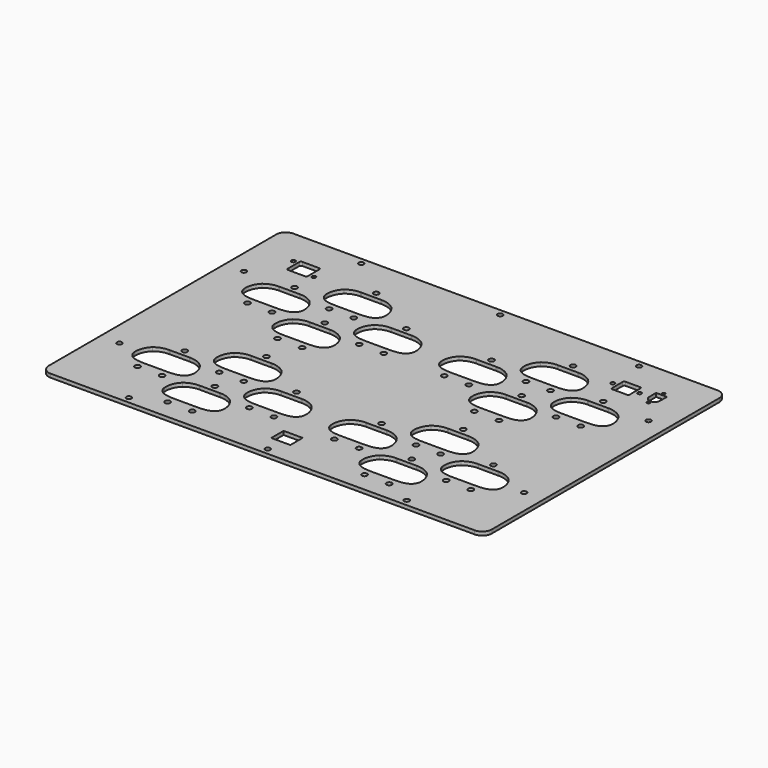
from build123d import *

# Parameters (mm, degrees)
F0_R     = 2.1
F0_R_2   = 2.2
F0_W     = 15.7
F0_H     = 12.7
F0_R_3   = 1.625
F0_R_4   = 1.6
F0_R_5   = 1.3
F1_DEPTH = 3


# Not quite as in the source:
# - the dataset's text gives a spline's control points without its knots; the knots are read off the source's solid


with BuildPart() as f1:
    # F0 (on Top) → F1 (new body)
    with BuildSketch(Plane.XY):
        with BuildLine():
            Line((174.5, 124.8), (-174.5, 124.8))
            ThreePointArc((-174.5, 124.8), (-180.0154328933, 122.5154328933), (-182.3, 117))
            Line((-182.3, 117), (-182.3, -117))
            ThreePointArc((-182.3, -117), (-180.0154328933, -122.5154328933), (-174.5, -124.8))
            Line((-174.5, -124.8), (174.5, -124.8))
            ThreePointArc((174.5, -124.8), (180.0154328933, -122.5154328933), (182.3, -117))
            Line((182.3, -117), (182.3, 117))
            ThreePointArc((182.3, 117), (180.0154328933, 122.5154328933), (174.5, 124.8))
        make_face()
        with Locations((-114.33, -119.5)):
            Circle(F0_R, mode=Mode.SUBTRACT)
        with Locations((-137.12, -82.102)):
            Circle(F0_R_2, mode=Mode.SUBTRACT)
        with Locations((-166.5, -64)):
            Circle(F0_R, mode=Mode.SUBTRACT)
        with Locations((-116.88, -82.102)):
            Circle(F0_R_2, mode=Mode.SUBTRACT)
        with BuildLine():
            Line((-135.6612948233, -51.451130735), (-135.115026498, -51.4620000001))
            Line((-135.115026498, -51.4620000001), (-118.8944121234, -51.4620000001))
            Line((-118.8944121234, -51.4620000001), (-118.3330315352, -51.4511211146))
            ThreePointArc((-118.3330315352, -51.4511211146), (-112.5954929046, -52.4136608229), (-107.487280821, -55.1979024679))
            ThreePointArc((-107.487280821, -55.1979024679), (-103.7289593809, -60.9649156398), (-102.7756384695, -67.7821438311))
            add(Edge.make_bspline(
                [(-102.7756384695, -67.7821438311), (-102.8317808557, -68.4791518436), (-103.1342622315, -69.8522558093), (-104.1227442667, -71.7376713061), (-105.3617732771, -73.0712234734), (-106.5853971676, -73.93803931), (-107.9464485907, -74.6539246569), (-109.8851336202, -75.2963766675), (-112.5588382079, -75.7473994177), (-115.5566427484, -75.9552688032), (-117.7556974045, -75.97825395), (-118.9009345935, -75.9720000001)],
                knots=[0, 0, 0, 0, 0.125, 0.25, 0.375, 0.4375, 0.5, 0.625, 0.75, 0.875, 0.9999501857, 0.9999501857, 0.9999501857, 0.9999501857], degree=3))
            Line((-118.9009345935, -75.9720000001), (-135.1072635354, -75.9720000001))
            Line((-135.1072635354, -75.9720000001), (-135.1086333173, -75.9720000001))
            add(Edge.make_bspline(
                [(-151.2339294072, -67.7821438309), (-151.177741554, -68.4797163167), (-150.8726831114, -69.8530561961), (-149.8774581613, -71.7367332364), (-148.6340002387, -73.0683891085), (-147.4094063644, -73.9344572306), (-146.0489657757, -74.6503376548), (-144.1131861346, -75.2935631846), (-141.4445788782, -75.7458922174), (-138.4515011772, -75.954911071), (-136.2539205452, -75.9782540848), (-135.1086333173, -75.9720000001)],
                knots=[0, 0, 0, 0, 0.125, 0.25, 0.375, 0.4375, 0.5, 0.625, 0.75, 0.875, 0.9999501867, 0.9999501867, 0.9999501867, 0.9999501867], degree=3))
            ThreePointArc((-151.2339294072, -67.7821438309), (-150.2806084958, -60.9649156397), (-146.5222870557, -55.1979024678))
            ThreePointArc((-146.5222870557, -55.1979024678), (-141.4068713777, -52.411174013), (-135.6612948233, -51.451130735))
        make_face(mode=Mode.SUBTRACT)
        with Locations((-91.12, -108.602)):
            Circle(F0_R_2, mode=Mode.SUBTRACT)
        with Locations((-70.88, -108.602)):
            Circle(F0_R_2, mode=Mode.SUBTRACT)
        with BuildLine():
            Line((-89.6612948233, -77.951130735), (-89.115026498, -77.9620000001))
            Line((-89.115026498, -77.9620000001), (-72.8944121234, -77.9620000001))
            Line((-72.8944121234, -77.9620000001), (-72.3330315352, -77.9511211146))
            ThreePointArc((-72.3330315352, -77.9511211146), (-66.5954929046, -78.9136608229), (-61.487280821, -81.6979024679))
            ThreePointArc((-61.487280821, -81.6979024679), (-57.7289593809, -87.4649156398), (-56.7756384695, -94.2821438311))
            add(Edge.make_bspline(
                [(-56.7756384695, -94.2821438311), (-56.8318288861, -94.9783630519), (-57.1341419789, -96.3506841544), (-58.1219861034, -98.2355446893), (-59.3608225377, -99.5692757568), (-60.5843212484, -100.4362682741), (-61.9452692843, -101.1523501476), (-63.8838615244, -101.7950820951), (-66.5575009571, -102.2464909201), (-69.5556737218, -102.4548208566), (-71.7552033004, -102.4781051534), (-72.9009345935, -102.4720000001)],
                knots=[0.0001387542, 0.0001387542, 0.0001387542, 0.0001387542, 0.125, 0.25, 0.375, 0.4375, 0.5, 0.625, 0.75, 0.875, 1, 1, 1, 1], degree=3))
            Line((-72.9009345935, -102.4720000001), (-89.1072635354, -102.4720000001))
            Line((-89.1072635354, -102.4720000001), (-89.1086333173, -102.4720000001))
            add(Edge.make_bspline(
                [(-105.2339294072, -94.2821438309), (-105.177741554, -94.9797163167), (-104.8726831114, -96.3530561961), (-103.8774581613, -98.2367332364), (-102.6340002387, -99.5683891085), (-101.4094063644, -100.4344572306), (-100.0489657757, -101.1503376548), (-98.1131861346, -101.7935631846), (-95.4445788782, -102.2458922174), (-92.4515011772, -102.454911071), (-90.2539205452, -102.4782540848), (-89.1086333173, -102.4720000001)],
                knots=[0, 0, 0, 0, 0.125, 0.25, 0.375, 0.4375, 0.5, 0.625, 0.75, 0.875, 0.9999501867, 0.9999501867, 0.9999501867, 0.9999501867], degree=3))
            ThreePointArc((-105.2339294072, -94.2821438309), (-104.2806084958, -87.4649156397), (-100.5222870557, -81.6979024678))
            ThreePointArc((-100.5222870557, -81.6979024678), (-95.4068713777, -78.911174013), (-89.6612948233, -77.951130735))
        make_face(mode=Mode.SUBTRACT)
        with Locations((-81, -72.692)):
            Circle(F0_R_2, mode=Mode.SUBTRACT)
        with Locations((-45.12, -82.102)):
            Circle(F0_R_2, mode=Mode.SUBTRACT)
        with Locations((-24.88, -82.102)):
            Circle(F0_R_2, mode=Mode.SUBTRACT)
        with BuildLine():
            Line((-43.6612948233, -51.451130735), (-43.115026498, -51.4620000001))
            Line((-43.115026498, -51.4620000001), (-26.8944121234, -51.4620000001))
            Line((-26.8944121234, -51.4620000001), (-26.3330315352, -51.4511211146))
            ThreePointArc((-26.3330315352, -51.4511211146), (-20.5954929046, -52.4136608229), (-15.487280821, -55.1979024679))
            ThreePointArc((-15.487280821, -55.1979024679), (-11.7289593809, -60.9649156398), (-10.7756384695, -67.7821438311))
            add(Edge.make_bspline(
                [(-10.7756384695, -67.7821438311), (-10.8317808557, -68.4791518436), (-11.1342622315, -69.8522558093), (-12.1227442667, -71.7376713061), (-13.3617732771, -73.0712234734), (-14.5853971676, -73.93803931), (-15.9464485907, -74.6539246569), (-17.8851336202, -75.2963766675), (-20.5588382079, -75.7473994177), (-23.5566427484, -75.9552688032), (-25.7556974045, -75.97825395), (-26.9009345935, -75.9720000001)],
                knots=[0, 0, 0, 0, 0.125, 0.25, 0.375, 0.4375, 0.5, 0.625, 0.75, 0.875, 0.9999501857, 0.9999501857, 0.9999501857, 0.9999501857], degree=3))
            Line((-26.9009345935, -75.9720000001), (-43.1072635354, -75.9720000001))
            Line((-43.1072635354, -75.9720000001), (-43.1086333173, -75.9720000001))
            add(Edge.make_bspline(
                [(-59.2339294072, -67.7821438309), (-59.177741554, -68.4797163167), (-58.8726831114, -69.8530561961), (-57.8774581613, -71.7367332364), (-56.6340002387, -73.0683891085), (-55.4094063644, -73.9344572306), (-54.0489657757, -74.6503376548), (-52.1131861346, -75.2935631846), (-49.4445788782, -75.7458922174), (-46.4515011772, -75.954911071), (-44.2539205452, -75.9782540848), (-43.1086333173, -75.9720000001)],
                knots=[0, 0, 0, 0, 0.125, 0.25, 0.375, 0.4375, 0.5, 0.625, 0.75, 0.875, 0.9999501867, 0.9999501867, 0.9999501867, 0.9999501867], degree=3))
            ThreePointArc((-59.2339294072, -67.7821438309), (-58.2806084958, -60.9649156397), (-54.5222870557, -55.1979024678))
            ThreePointArc((-54.5222870557, -55.1979024678), (-49.4068713777, -52.411174013), (-43.6612948233, -51.451130735))
        make_face(mode=Mode.SUBTRACT)
        with Locations((-127, -46.192)):
            Circle(F0_R_2, mode=Mode.SUBTRACT)
        with Locations((-91.12, -55.602)):
            Circle(F0_R_2, mode=Mode.SUBTRACT)
        with Locations((-70.88, -55.602)):
            Circle(F0_R_2, mode=Mode.SUBTRACT)
        with BuildLine():
            Line((-89.6612948233, -24.951130735), (-89.115026498, -24.9620000001))
            Line((-89.115026498, -24.9620000001), (-72.8944121234, -24.9620000001))
            Line((-72.8944121234, -24.9620000001), (-72.3330315352, -24.9511211146))
            ThreePointArc((-72.3330315352, -24.9511211146), (-66.5954929046, -25.9136608229), (-61.487280821, -28.6979024679))
            ThreePointArc((-61.487280821, -28.6979024679), (-57.7289593809, -34.4649156398), (-56.7756384695, -41.2821438311))
            add(Edge.make_bspline(
                [(-56.7756384695, -41.2821438311), (-56.8317808557, -41.9791518436), (-57.1342622315, -43.3522558093), (-58.1227442667, -45.2376713061), (-59.3617732771, -46.5712234734), (-60.5853971676, -47.43803931), (-61.9464485907, -48.1539246569), (-63.8851336202, -48.7963766675), (-66.5588382079, -49.2473994177), (-69.5566427484, -49.4552688032), (-71.7556974045, -49.47825395), (-72.9009345935, -49.4720000001)],
                knots=[0, 0, 0, 0, 0.125, 0.25, 0.375, 0.4375, 0.5, 0.625, 0.75, 0.875, 0.9999501857, 0.9999501857, 0.9999501857, 0.9999501857], degree=3))
            Line((-72.9009345935, -49.4720000001), (-89.1072635354, -49.4720000001))
            Line((-89.1072635354, -49.4720000001), (-89.1086333173, -49.4720000001))
            add(Edge.make_bspline(
                [(-105.2339294072, -41.2821438309), (-105.177741554, -41.9797163167), (-104.8726831114, -43.3530561961), (-103.8774581613, -45.2367332364), (-102.6340002387, -46.5683891085), (-101.4094063644, -47.4344572306), (-100.0489657757, -48.1503376548), (-98.1131861346, -48.7935631846), (-95.4445788782, -49.2458922174), (-92.4515011772, -49.454911071), (-90.2539205452, -49.4782540848), (-89.1086333173, -49.4720000001)],
                knots=[0, 0, 0, 0, 0.125, 0.25, 0.375, 0.4375, 0.5, 0.625, 0.75, 0.875, 0.9999501867, 0.9999501867, 0.9999501867, 0.9999501867], degree=3))
            ThreePointArc((-105.2339294072, -41.2821438309), (-104.2806084958, -34.4649156397), (-100.5222870557, -28.6979024678))
            ThreePointArc((-100.5222870557, -28.6979024678), (-95.4068713777, -25.911174013), (-89.6612948233, -24.951130735))
        make_face(mode=Mode.SUBTRACT)
        with Locations((-35, -46.192)):
            Circle(F0_R_2, mode=Mode.SUBTRACT)
        with Locations((-81, -19.692)):
            Circle(F0_R_2, mode=Mode.SUBTRACT)
        with Locations((0, -119.5)):
            Circle(F0_R, mode=Mode.SUBTRACT)
        with Locations((0, -99.8)):
            Rectangle(F0_W, F0_H, mode=Mode.SUBTRACT)
        with Locations((70.88, -108.602)):
            Circle(F0_R_2, mode=Mode.SUBTRACT)
        with Locations((91.12, -108.602)):
            Circle(F0_R_2, mode=Mode.SUBTRACT)
        with Locations((24.88, -82.102)):
            Circle(F0_R_2, mode=Mode.SUBTRACT)
        with Locations((45.12, -82.102)):
            Circle(F0_R_2, mode=Mode.SUBTRACT)
        with BuildLine():
            Line((26.3387051767, -51.451130735), (26.884973502, -51.4620000001))
            Line((26.884973502, -51.4620000001), (43.1055878766, -51.4620000001))
            Line((43.1055878766, -51.4620000001), (43.6669684648, -51.4511211146))
            ThreePointArc((43.6669684648, -51.4511211146), (49.4045070954, -52.4136608229), (54.512719179, -55.1979024679))
            ThreePointArc((54.512719179, -55.1979024679), (58.2710406191, -60.9649156398), (59.2243615305, -67.7821438311))
            add(Edge.make_bspline(
                [(59.2243615305, -67.7821438311), (59.1682191443, -68.4791518436), (58.8657377685, -69.8522558093), (57.8772557333, -71.7376713061), (56.6382267229, -73.0712234734), (55.4146028324, -73.93803931), (54.0535514093, -74.6539246569), (52.1148663798, -75.2963766675), (49.4411617921, -75.7473994177), (46.4433572516, -75.9552688032), (44.2443025955, -75.97825395), (43.0990654065, -75.9720000001)],
                knots=[0, 0, 0, 0, 0.125, 0.25, 0.375, 0.4375, 0.5, 0.625, 0.75, 0.875, 0.9999501857, 0.9999501857, 0.9999501857, 0.9999501857], degree=3))
            Line((43.0990654065, -75.9720000001), (26.8927364646, -75.9720000001))
            Line((26.8927364646, -75.9720000001), (26.8913666827, -75.9720000001))
            add(Edge.make_bspline(
                [(10.7660705928, -67.7821438309), (10.822258446, -68.4797163167), (11.1273168886, -69.8530561961), (12.1225418387, -71.7367332364), (13.3659997613, -73.0683891085), (14.5905936356, -73.9344572306), (15.9510342243, -74.6503376548), (17.8868138654, -75.2935631846), (20.5554211218, -75.7458922174), (23.5484988228, -75.954911071), (25.7460794548, -75.9782540848), (26.8913666827, -75.9720000001)],
                knots=[0, 0, 0, 0, 0.125, 0.25, 0.375, 0.4375, 0.5, 0.625, 0.75, 0.875, 0.9999501867, 0.9999501867, 0.9999501867, 0.9999501867], degree=3))
            ThreePointArc((10.7660705928, -67.7821438309), (11.7193915042, -60.9649156397), (15.4777129443, -55.1979024678))
            ThreePointArc((15.4777129443, -55.1979024678), (20.5931286223, -52.411174013), (26.3387051767, -51.451130735))
        make_face(mode=Mode.SUBTRACT)
        with BuildLine():
            Line((72.3387051767, -77.951130735), (72.884973502, -77.9620000001))
            Line((72.884973502, -77.9620000001), (89.1055878766, -77.9620000001))
            Line((89.1055878766, -77.9620000001), (89.6669684648, -77.9511211146))
            ThreePointArc((89.6669684648, -77.9511211146), (95.4045070954, -78.9136608229), (100.512719179, -81.6979024679))
            ThreePointArc((100.512719179, -81.6979024679), (104.2710406191, -87.4649156398), (105.2243615305, -94.2821438311))
            add(Edge.make_bspline(
                [(105.2243615305, -94.2821438311), (105.1682191443, -94.9791518436), (104.8657377685, -96.3522558093), (103.8772557333, -98.2376713061), (102.6382267229, -99.5712234734), (101.4146028324, -100.43803931), (100.0535514093, -101.1539246569), (98.1148663798, -101.7963766675), (95.4411617921, -102.2473994177), (92.4433572516, -102.4552688032), (90.2443025955, -102.47825395), (89.0990654065, -102.4720000001)],
                knots=[0, 0, 0, 0, 0.125, 0.25, 0.375, 0.4375, 0.5, 0.625, 0.75, 0.875, 0.9999501857, 0.9999501857, 0.9999501857, 0.9999501857], degree=3))
            Line((89.0990654065, -102.4720000001), (72.8927364646, -102.4720000001))
            Line((72.8927364646, -102.4720000001), (72.8913666827, -102.4720000001))
            add(Edge.make_bspline(
                [(56.7660705928, -94.2821438309), (56.822258446, -94.9797163167), (57.1273168886, -96.3530561961), (58.1225418387, -98.2367332364), (59.3659997613, -99.5683891085), (60.5905936356, -100.4344572306), (61.9510342243, -101.1503376548), (63.8868138654, -101.7935631846), (66.5554211218, -102.2458922174), (69.5484988228, -102.454911071), (71.7460794548, -102.4782540848), (72.8913666827, -102.4720000001)],
                knots=[0, 0, 0, 0, 0.125, 0.25, 0.375, 0.4375, 0.5, 0.625, 0.75, 0.875, 0.9999501867, 0.9999501867, 0.9999501867, 0.9999501867], degree=3))
            ThreePointArc((56.7660705928, -94.2821438309), (57.7193915042, -87.4649156397), (61.4777129443, -81.6979024678))
            ThreePointArc((61.4777129443, -81.6979024678), (66.5931286223, -78.911174013), (72.3387051767, -77.951130735))
        make_face(mode=Mode.SUBTRACT)
        with Locations((81, -72.692)):
            Circle(F0_R_2, mode=Mode.SUBTRACT)
        with Locations((114.33, -119.5)):
            Circle(F0_R, mode=Mode.SUBTRACT)
        with Locations((116.88, -82.102)):
            Circle(F0_R_2, mode=Mode.SUBTRACT)
        with BuildLine():
            Line((118.3387051767, -51.451130735), (118.884973502, -51.4620000001))
            Line((118.884973502, -51.4620000001), (135.1055878766, -51.4620000001))
            Line((135.1055878766, -51.4620000001), (135.6669684648, -51.4511211146))
            ThreePointArc((135.6669684648, -51.4511211146), (141.4045070954, -52.4136608229), (146.512719179, -55.1979024679))
            ThreePointArc((146.512719179, -55.1979024679), (150.2710406191, -60.9649156398), (151.2243615305, -67.7821438311))
            add(Edge.make_bspline(
                [(151.2243615305, -67.7821438311), (151.1682191443, -68.4791518436), (150.8657377685, -69.8522558093), (149.8772557333, -71.7376713061), (148.6382267229, -73.0712234734), (147.4146028324, -73.93803931), (146.0535514093, -74.6539246569), (144.1148663798, -75.2963766675), (141.4411617921, -75.7473994177), (138.4433572516, -75.9552688032), (136.2443025955, -75.97825395), (135.0990654065, -75.9720000001)],
                knots=[0, 0, 0, 0, 0.125, 0.25, 0.375, 0.4375, 0.5, 0.625, 0.75, 0.875, 0.9999501857, 0.9999501857, 0.9999501857, 0.9999501857], degree=3))
            Line((135.0990654065, -75.9720000001), (118.8927364646, -75.9720000001))
            Line((118.8927364646, -75.9720000001), (118.8913666827, -75.9720000001))
            add(Edge.make_bspline(
                [(102.7660705928, -67.7821438309), (102.822258446, -68.4797163167), (103.1273168886, -69.8530561961), (104.1225418387, -71.7367332364), (105.3659997613, -73.0683891085), (106.5905936356, -73.9344572306), (107.9510342243, -74.6503376548), (109.8868138654, -75.2935631846), (112.5554211218, -75.7458922174), (115.5484988228, -75.954911071), (117.7460794548, -75.9782540848), (118.8913666827, -75.9720000001)],
                knots=[0, 0, 0, 0, 0.125, 0.25, 0.375, 0.4375, 0.5, 0.625, 0.75, 0.875, 0.9999501867, 0.9999501867, 0.9999501867, 0.9999501867], degree=3))
            ThreePointArc((102.7660705928, -67.7821438309), (103.7193915042, -60.9649156397), (107.4777129443, -55.1979024678))
            ThreePointArc((107.4777129443, -55.1979024678), (112.5931286223, -52.411174013), (118.3387051767, -51.451130735))
        make_face(mode=Mode.SUBTRACT)
        with Locations((137.12, -82.102)):
            Circle(F0_R_2, mode=Mode.SUBTRACT)
        with Locations((166.5, -64)):
            Circle(F0_R, mode=Mode.SUBTRACT)
        with Locations((35, -46.192)):
            Circle(F0_R_2, mode=Mode.SUBTRACT)
        with Locations((70.88, -55.602)):
            Circle(F0_R_2, mode=Mode.SUBTRACT)
        with Locations((91.12, -55.602)):
            Circle(F0_R_2, mode=Mode.SUBTRACT)
        with BuildLine():
            Line((72.3387051767, -24.951130735), (72.884973502, -24.9620000001))
            Line((72.884973502, -24.9620000001), (89.1055878766, -24.9620000001))
            Line((89.1055878766, -24.9620000001), (89.6669684648, -24.9511211146))
            ThreePointArc((89.6669684648, -24.9511211146), (95.4045070954, -25.9136608229), (100.512719179, -28.6979024679))
            ThreePointArc((100.512719179, -28.6979024679), (104.2710406191, -34.4649156398), (105.2243615305, -41.2821438311))
            add(Edge.make_bspline(
                [(105.2243615305, -41.2821438311), (105.1682191443, -41.9791518436), (104.8657377685, -43.3522558093), (103.8772557333, -45.2376713061), (102.6382267229, -46.5712234734), (101.4146028324, -47.43803931), (100.0535514093, -48.1539246569), (98.1148663798, -48.7963766675), (95.4411617921, -49.2473994177), (92.4433572516, -49.4552688032), (90.2443025955, -49.47825395), (89.0990654065, -49.4720000001)],
                knots=[0, 0, 0, 0, 0.125, 0.25, 0.375, 0.4375, 0.5, 0.625, 0.75, 0.875, 0.9999501857, 0.9999501857, 0.9999501857, 0.9999501857], degree=3))
            Line((89.0990654065, -49.4720000001), (72.8927364646, -49.4720000001))
            Line((72.8927364646, -49.4720000001), (72.8913666827, -49.4720000001))
            add(Edge.make_bspline(
                [(56.7660705928, -41.2821438309), (56.822258446, -41.9797163167), (57.1273168886, -43.3530561961), (58.1225418387, -45.2367332364), (59.3659997613, -46.5683891085), (60.5905936356, -47.4344572306), (61.9510342243, -48.1503376548), (63.8868138654, -48.7935631846), (66.5554211218, -49.2458922174), (69.5484988228, -49.454911071), (71.7460794548, -49.4782540848), (72.8913666827, -49.4720000001)],
                knots=[0, 0, 0, 0, 0.125, 0.25, 0.375, 0.4375, 0.5, 0.625, 0.75, 0.875, 0.9999501867, 0.9999501867, 0.9999501867, 0.9999501867], degree=3))
            ThreePointArc((56.7660705928, -41.2821438309), (57.7193915042, -34.4649156397), (61.4777129443, -28.6979024678))
            ThreePointArc((61.4777129443, -28.6979024678), (66.5931286223, -25.911174013), (72.3387051767, -24.951130735))
        make_face(mode=Mode.SUBTRACT)
        with Locations((81, -19.692)):
            Circle(F0_R_2, mode=Mode.SUBTRACT)
        with Locations((127, -46.192)):
            Circle(F0_R_2, mode=Mode.SUBTRACT)
        with Locations((-137.12, 30.898)):
            Circle(F0_R_2, mode=Mode.SUBTRACT)
        with Locations((-116.88, 30.898)):
            Circle(F0_R_2, mode=Mode.SUBTRACT)
        with BuildLine():
            Line((-135.6612948233, 61.548869265), (-135.115026498, 61.5379999999))
            Line((-135.115026498, 61.5379999999), (-118.8944121234, 61.5379999999))
            Line((-118.8944121234, 61.5379999999), (-118.3330315352, 61.5488788854))
            ThreePointArc((-118.3330315352, 61.5488788854), (-112.5954929046, 60.5863391771), (-107.487280821, 57.8020975321))
            ThreePointArc((-107.487280821, 57.8020975321), (-103.7289593809, 52.0350843602), (-102.7756384695, 45.2178561689))
            add(Edge.make_bspline(
                [(-102.7756384695, 45.2178561689), (-102.8317808557, 44.5208481564), (-103.1342622315, 43.1477441907), (-104.1227442667, 41.2623286939), (-105.3617732771, 39.9287765266), (-106.5853971676, 39.06196069), (-107.9464485907, 38.3460753431), (-109.8851336202, 37.7036233325), (-112.5588382079, 37.2526005823), (-115.5566427484, 37.0447311968), (-117.7556974045, 37.02174605), (-118.9009345935, 37.0279999999)],
                knots=[0, 0, 0, 0, 0.125, 0.25, 0.375, 0.4375, 0.5, 0.625, 0.75, 0.875, 0.9999501857, 0.9999501857, 0.9999501857, 0.9999501857], degree=3))
            Line((-118.9009345935, 37.0279999999), (-135.1072635354, 37.0279999999))
            Line((-135.1072635354, 37.0279999999), (-135.1086333173, 37.0279999999))
            add(Edge.make_bspline(
                [(-151.2339294072, 45.2178561691), (-151.177741554, 44.5202836833), (-150.8726831114, 43.1469438039), (-149.8774581613, 41.2632667636), (-148.6340002387, 39.9316108915), (-147.4094063644, 39.0655427694), (-146.0489657757, 38.3496623452), (-144.1131861346, 37.7064368154), (-141.4445788782, 37.2541077826), (-138.4515011772, 37.045088929), (-136.2539205452, 37.0217459152), (-135.1086333173, 37.0279999999)],
                knots=[0, 0, 0, 0, 0.125, 0.25, 0.375, 0.4375, 0.5, 0.625, 0.75, 0.875, 0.9999501867, 0.9999501867, 0.9999501867, 0.9999501867], degree=3))
            ThreePointArc((-151.2339294072, 45.2178561691), (-150.2806084958, 52.0350843603), (-146.5222870557, 57.8020975322))
            ThreePointArc((-146.5222870557, 57.8020975322), (-141.4068713777, 60.588825987), (-135.6612948233, 61.548869265))
        make_face(mode=Mode.SUBTRACT)
        with Locations((-91.12, 4.398)):
            Circle(F0_R_2, mode=Mode.SUBTRACT)
        with Locations((-70.88, 4.398)):
            Circle(F0_R_2, mode=Mode.SUBTRACT)
        with BuildLine():
            Line((-89.6612948233, 35.048869265), (-89.115026498, 35.0379999999))
            Line((-89.115026498, 35.0379999999), (-72.8944121234, 35.0379999999))
            Line((-72.8944121234, 35.0379999999), (-72.3330315352, 35.0488788854))
            ThreePointArc((-72.3330315352, 35.0488788854), (-66.5954929046, 34.0863391771), (-61.487280821, 31.3020975321))
            ThreePointArc((-61.487280821, 31.3020975321), (-57.7289593809, 25.5350843602), (-56.7756384695, 18.7178561689))
            add(Edge.make_bspline(
                [(-56.7756384695, 18.7178561689), (-56.8317808557, 18.0208481564), (-57.1342622315, 16.6477441907), (-58.1227442667, 14.7623286939), (-59.3617732771, 13.4287765266), (-60.5853971676, 12.56196069), (-61.9464485907, 11.8460753431), (-63.8851336202, 11.2036233325), (-66.5588382079, 10.7526005823), (-69.5566427484, 10.5447311968), (-71.7556974045, 10.52174605), (-72.9009345935, 10.5279999999)],
                knots=[0, 0, 0, 0, 0.125, 0.25, 0.375, 0.4375, 0.5, 0.625, 0.75, 0.875, 0.9999501857, 0.9999501857, 0.9999501857, 0.9999501857], degree=3))
            Line((-72.9009345935, 10.5279999999), (-89.1072635354, 10.5279999999))
            Line((-89.1072635354, 10.5279999999), (-89.1086333173, 10.5279999999))
            add(Edge.make_bspline(
                [(-105.2339294072, 18.7178561691), (-105.177741554, 18.0202836833), (-104.8726831114, 16.6469438039), (-103.8774581613, 14.7632667636), (-102.6340002387, 13.4316108915), (-101.4094063644, 12.5655427694), (-100.0489657757, 11.8496623452), (-98.1131861346, 11.2064368154), (-95.4445788782, 10.7541077826), (-92.4515011772, 10.545088929), (-90.2539205452, 10.5217459152), (-89.1086333173, 10.5279999999)],
                knots=[0, 0, 0, 0, 0.125, 0.25, 0.375, 0.4375, 0.5, 0.625, 0.75, 0.875, 0.9999501867, 0.9999501867, 0.9999501867, 0.9999501867], degree=3))
            ThreePointArc((-105.2339294072, 18.7178561691), (-104.2806084958, 25.5350843603), (-100.5222870557, 31.3020975322))
            ThreePointArc((-100.5222870557, 31.3020975322), (-95.4068713777, 34.088825987), (-89.6612948233, 35.048869265))
        make_face(mode=Mode.SUBTRACT)
        with Locations((-45.12, 30.898)):
            Circle(F0_R_2, mode=Mode.SUBTRACT)
        with Locations((-24.88, 30.898)):
            Circle(F0_R_2, mode=Mode.SUBTRACT)
        with Locations((-81, 40.308)):
            Circle(F0_R_2, mode=Mode.SUBTRACT)
        with Locations((-91.12, 57.398)):
            Circle(F0_R_2, mode=Mode.SUBTRACT)
        with Locations((-70.88, 57.398)):
            Circle(F0_R_2, mode=Mode.SUBTRACT)
        with BuildLine():
            Line((-43.6612948233, 61.548869265), (-43.115026498, 61.5379999999))
            Line((-43.115026498, 61.5379999999), (-26.8944121234, 61.5379999999))
            Line((-26.8944121234, 61.5379999999), (-26.3330315352, 61.5488788854))
            ThreePointArc((-26.3330315352, 61.5488788854), (-20.5954929046, 60.5863391771), (-15.487280821, 57.8020975321))
            ThreePointArc((-15.487280821, 57.8020975321), (-11.7282191214, 52.0352577574), (-10.7742686876, 45.2178561689))
            add(Edge.make_bspline(
                [(-10.7742686876, 45.2178561689), (-10.8304110738, 44.5208481564), (-11.1328924496, 43.1477441907), (-12.1213744847, 41.2623286939), (-13.3604034952, 39.9287765266), (-14.5840273857, 39.06196069), (-15.9450788087, 38.3460753431), (-17.8837638383, 37.7036233325), (-20.557468426, 37.2526005823), (-23.5552729664, 37.0447311968), (-25.7543276226, 37.02174605), (-26.8995648116, 37.0279999999)],
                knots=[0, 0, 0, 0, 0.125, 0.25, 0.375, 0.4375, 0.5, 0.625, 0.75, 0.875, 0.9999501857, 0.9999501857, 0.9999501857, 0.9999501857], degree=3))
            Line((-26.8995648116, 37.0279999999), (-43.1072635354, 37.0279999999))
            add(Edge.make_bspline(
                [(-59.2325596253, 45.2178561691), (-59.1763212388, 44.5210734563), (-58.8714315071, 43.1485163208), (-57.876846428, 41.2653920745), (-56.633580812, 39.9335566586), (-55.4091120122, 39.0673117119), (-54.0487748122, 38.3512348451), (-52.1130880742, 37.7077297918), (-49.4445461628, 37.255015412), (-46.4511010398, 37.0455365283), (-44.2530455057, 37.0218945801), (-43.1072635354, 37.0279999999)],
                knots=[0.0001386451, 0.0001386451, 0.0001386451, 0.0001386451, 0.125, 0.25, 0.375, 0.4375, 0.5, 0.625, 0.75, 0.875, 1, 1, 1, 1], degree=3))
            ThreePointArc((-59.2325596253, 45.2178561691), (-58.2798682404, 52.0349109767), (-54.5222870557, 57.8020975322))
            ThreePointArc((-54.5222870557, 57.8020975322), (-49.4068713777, 60.588825987), (-43.6612948233, 61.548869265))
        make_face(mode=Mode.SUBTRACT)
        with Locations((-166.5, 64)):
            Circle(F0_R, mode=Mode.SUBTRACT)
        with BuildLine():
            ThreePointArc((-146.775, 96.295), (-146.370807358, 97.270807358), (-145.395, 97.675))
            Line((-145.395, 97.675), (-131.605, 97.675))
            ThreePointArc((-131.605, 97.675), (-130.629192642, 97.270807358), (-130.225, 96.295))
            Line((-130.225, 96.295), (-130.225, 84.505))
            ThreePointArc((-130.225, 84.505), (-130.629192642, 83.529192642), (-131.605, 83.125))
            Line((-131.605, 83.125), (-145.395, 83.125))
            ThreePointArc((-145.395, 83.125), (-146.370807358, 83.529192642), (-146.775, 84.505))
            Line((-146.775, 84.505), (-146.775, 96.295))
        make_face(mode=Mode.SUBTRACT)
        with Locations((-127, 66.808)):
            Circle(F0_R_2, mode=Mode.SUBTRACT)
        with Locations((-126.5, 85.9)):
            Circle(F0_R_3, mode=Mode.SUBTRACT)
        with Locations((-150.5, 94.9)):
            Circle(F0_R_3, mode=Mode.SUBTRACT)
        with Locations((-114.33, 119.5)):
            Circle(F0_R, mode=Mode.SUBTRACT)
        with BuildLine():
            Line((-89.6612948233, 88.048869265), (-89.115026498, 88.0379999999))
            Line((-89.115026498, 88.0379999999), (-72.8944121234, 88.0379999999))
            Line((-72.8944121234, 88.0379999999), (-72.3330315352, 88.0488788854))
            ThreePointArc((-72.3330315352, 88.0488788854), (-66.5954929046, 87.0863391771), (-61.487280821, 84.3020975321))
            ThreePointArc((-61.487280821, 84.3020975321), (-57.7289593809, 78.5350843602), (-56.7756384695, 71.7178561689))
            add(Edge.make_bspline(
                [(-56.7756384695, 71.7178561689), (-56.8317808557, 71.0208481564), (-57.1342622315, 69.6477441907), (-58.1227442667, 67.7623286939), (-59.3617732771, 66.4287765266), (-60.5853971676, 65.56196069), (-61.9464485907, 64.8460753431), (-63.8851336202, 64.2036233325), (-66.5588382079, 63.7526005823), (-69.5566427484, 63.5447311968), (-71.7556974045, 63.52174605), (-72.9009345935, 63.5279999999)],
                knots=[0, 0, 0, 0, 0.125, 0.25, 0.375, 0.4375, 0.5, 0.625, 0.75, 0.875, 0.9999501857, 0.9999501857, 0.9999501857, 0.9999501857], degree=3))
            Line((-72.9009345935, 63.5279999999), (-89.1072635354, 63.5279999999))
            Line((-89.1072635354, 63.5279999999), (-89.1086333173, 63.5279999999))
            add(Edge.make_bspline(
                [(-105.2339294072, 71.7178561691), (-105.177741554, 71.0202836833), (-104.8726831114, 69.6469438039), (-103.8774581613, 67.7632667636), (-102.6340002387, 66.4316108915), (-101.4094063644, 65.5655427694), (-100.0489657757, 64.8496623452), (-98.1131861346, 64.2064368154), (-95.4445788782, 63.7541077826), (-92.4515011772, 63.545088929), (-90.2539205452, 63.5217459152), (-89.1086333173, 63.5279999999)],
                knots=[0, 0, 0, 0, 0.125, 0.25, 0.375, 0.4375, 0.5, 0.625, 0.75, 0.875, 0.9999501867, 0.9999501867, 0.9999501867, 0.9999501867], degree=3))
            ThreePointArc((-105.2339294072, 71.7178561691), (-104.2806084958, 78.5350843603), (-100.5222870557, 84.3020975322))
            ThreePointArc((-100.5222870557, 84.3020975322), (-95.4068713777, 87.088825987), (-89.6612948233, 88.048869265))
        make_face(mode=Mode.SUBTRACT)
        with Locations((-81, 93.308)):
            Circle(F0_R_2, mode=Mode.SUBTRACT)
        with Locations((-35, 66.808)):
            Circle(F0_R_2, mode=Mode.SUBTRACT)
        with Locations((24.88, 30.898)):
            Circle(F0_R_2, mode=Mode.SUBTRACT)
        with Locations((45.12, 30.898)):
            Circle(F0_R_2, mode=Mode.SUBTRACT)
        with Locations((70.88, 4.398)):
            Circle(F0_R_2, mode=Mode.SUBTRACT)
        with Locations((91.12, 4.398)):
            Circle(F0_R_2, mode=Mode.SUBTRACT)
        with BuildLine():
            Line((72.3387051767, 35.048869265), (72.884973502, 35.0379999999))
            Line((72.884973502, 35.0379999999), (89.1055878766, 35.0379999999))
            Line((89.1055878766, 35.0379999999), (89.6669684648, 35.0488788854))
            ThreePointArc((89.6669684648, 35.0488788854), (95.4045070954, 34.0863391771), (100.512719179, 31.3020975321))
            ThreePointArc((100.512719179, 31.3020975321), (104.2710406191, 25.5350843602), (105.2243615305, 18.7178561689))
            add(Edge.make_bspline(
                [(105.2243615305, 18.7178561689), (105.1681711139, 18.0216369481), (104.8658580211, 16.6493158456), (103.8780138966, 14.7644553107), (102.6391774623, 13.4307242432), (101.4156787516, 12.5637317259), (100.0547307157, 11.8476498524), (98.1161384756, 11.2049179049), (95.4424990429, 10.7535090799), (92.4443262782, 10.5451791434), (90.2447966996, 10.5218948466), (89.0990654065, 10.5279999999)],
                knots=[0.0001387542, 0.0001387542, 0.0001387542, 0.0001387542, 0.125, 0.25, 0.375, 0.4375, 0.5, 0.625, 0.75, 0.875, 1, 1, 1, 1], degree=3))
            Line((89.0990654065, 10.5279999999), (72.8927364646, 10.5279999999))
            Line((72.8927364646, 10.5279999999), (72.8913666827, 10.5279999999))
            add(Edge.make_bspline(
                [(56.7660705928, 18.7178561691), (56.822258446, 18.0202836833), (57.1273168886, 16.6469438039), (58.1225418387, 14.7632667636), (59.3659997613, 13.4316108915), (60.5905936356, 12.5655427694), (61.9510342243, 11.8496623452), (63.8868138654, 11.2064368154), (66.5554211218, 10.7541077826), (69.5484988228, 10.545088929), (71.7460794548, 10.5217459152), (72.8913666827, 10.5279999999)],
                knots=[0, 0, 0, 0, 0.125, 0.25, 0.375, 0.4375, 0.5, 0.625, 0.75, 0.875, 0.9999501867, 0.9999501867, 0.9999501867, 0.9999501867], degree=3))
            ThreePointArc((56.7660705928, 18.7178561691), (57.7193915042, 25.5350843603), (61.4777129443, 31.3020975322))
            ThreePointArc((61.4777129443, 31.3020975322), (66.5931286223, 34.088825987), (72.3387051767, 35.048869265))
        make_face(mode=Mode.SUBTRACT)
        with BuildLine():
            Line((26.3387051767, 61.548869265), (26.884973502, 61.5379999999))
            Line((26.884973502, 61.5379999999), (43.1055878766, 61.5379999999))
            Line((43.1055878766, 61.5379999999), (43.6669684648, 61.5488788854))
            ThreePointArc((43.6669684648, 61.5488788854), (49.4045070954, 60.5863391771), (54.512719179, 57.8020975321))
            ThreePointArc((54.512719179, 57.8020975321), (58.2710406191, 52.0350843602), (59.2243615305, 45.2178561689))
            add(Edge.make_bspline(
                [(59.2243615305, 45.2178561689), (59.1681711139, 44.5216369481), (58.8658580211, 43.1493158456), (57.8780138966, 41.2644553107), (56.6391774623, 39.9307242432), (55.4156787516, 39.0637317259), (54.0547307157, 38.3476498524), (52.1161384756, 37.7049179049), (49.4424990429, 37.2535090799), (46.4443262782, 37.0451791434), (44.2447966996, 37.0218948466), (43.0990654065, 37.0279999999)],
                knots=[0.0001387542, 0.0001387542, 0.0001387542, 0.0001387542, 0.125, 0.25, 0.375, 0.4375, 0.5, 0.625, 0.75, 0.875, 1, 1, 1, 1], degree=3))
            Line((43.0990654065, 37.0279999999), (26.8927364646, 37.0279999999))
            Line((26.8927364646, 37.0279999999), (26.8913666827, 37.0279999999))
            add(Edge.make_bspline(
                [(10.7660705928, 45.2178561691), (10.822258446, 44.5202836833), (11.1273168886, 43.1469438039), (12.1225418387, 41.2632667636), (13.3659997613, 39.9316108915), (14.5905936356, 39.0655427694), (15.9510342243, 38.3496623452), (17.8868138654, 37.7064368154), (20.5554211218, 37.2541077826), (23.5484988228, 37.045088929), (25.7460794548, 37.0217459152), (26.8913666827, 37.0279999999)],
                knots=[0, 0, 0, 0, 0.125, 0.25, 0.375, 0.4375, 0.5, 0.625, 0.75, 0.875, 0.9999501867, 0.9999501867, 0.9999501867, 0.9999501867], degree=3))
            ThreePointArc((10.7660705928, 45.2178561691), (11.7193915042, 52.0350843603), (15.4777129443, 57.8020975322))
            ThreePointArc((15.4777129443, 57.8020975322), (20.5931286223, 60.588825987), (26.3387051767, 61.548869265))
        make_face(mode=Mode.SUBTRACT)
        with Locations((81, 40.308)):
            Circle(F0_R_2, mode=Mode.SUBTRACT)
        with Locations((70.88, 57.398)):
            Circle(F0_R_2, mode=Mode.SUBTRACT)
        with Locations((91.12, 57.398)):
            Circle(F0_R_2, mode=Mode.SUBTRACT)
        with Locations((116.88, 30.898)):
            Circle(F0_R_2, mode=Mode.SUBTRACT)
        with Locations((137.12, 30.898)):
            Circle(F0_R_2, mode=Mode.SUBTRACT)
        with BuildLine():
            Line((118.3387051767, 61.548869265), (118.884973502, 61.5379999999))
            Line((118.884973502, 61.5379999999), (135.1055878766, 61.5379999999))
            Line((135.1055878766, 61.5379999999), (135.6669684648, 61.5488788854))
            ThreePointArc((135.6669684648, 61.5488788854), (141.4045070954, 60.5863391771), (146.512719179, 57.8020975321))
            ThreePointArc((146.512719179, 57.8020975321), (150.2710406191, 52.0350843602), (151.2243615305, 45.2178561689))
            add(Edge.make_bspline(
                [(151.2243615305, 45.2178561689), (151.1681711139, 44.5216369481), (150.8658580211, 43.1493158456), (149.8780138966, 41.2644553107), (148.6391774623, 39.9307242432), (147.4156787516, 39.0637317259), (146.0547307157, 38.3476498524), (144.1161384756, 37.7049179049), (141.4424990429, 37.2535090799), (138.4443262782, 37.0451791434), (136.2447966996, 37.0218948466), (135.0990654065, 37.0279999999)],
                knots=[0.0001387542, 0.0001387542, 0.0001387542, 0.0001387542, 0.125, 0.25, 0.375, 0.4375, 0.5, 0.625, 0.75, 0.875, 1, 1, 1, 1], degree=3))
            Line((135.0990654065, 37.0279999999), (118.8927364646, 37.0279999999))
            Line((118.8927364646, 37.0279999999), (118.8913666827, 37.0279999999))
            add(Edge.make_bspline(
                [(102.7660705928, 45.2178561691), (102.822258446, 44.5202836833), (103.1273168886, 43.1469438039), (104.1225418387, 41.2632667636), (105.3659997613, 39.9316108915), (106.5905936356, 39.0655427694), (107.9510342243, 38.3496623452), (109.8868138654, 37.7064368154), (112.5554211218, 37.2541077826), (115.5484988228, 37.045088929), (117.7460794548, 37.0217459152), (118.8913666827, 37.0279999999)],
                knots=[0, 0, 0, 0, 0.125, 0.25, 0.375, 0.4375, 0.5, 0.625, 0.75, 0.875, 0.9999501867, 0.9999501867, 0.9999501867, 0.9999501867], degree=3))
            ThreePointArc((102.7660705928, 45.2178561691), (103.7193915042, 52.0350843603), (107.4777129443, 57.8020975322))
            ThreePointArc((107.4777129443, 57.8020975322), (112.5931286223, 60.588825987), (118.3387051767, 61.548869265))
        make_face(mode=Mode.SUBTRACT)
        with Locations((35, 66.808)):
            Circle(F0_R_2, mode=Mode.SUBTRACT)
        with BuildLine():
            Line((72.3387051767, 88.048869265), (72.884973502, 88.0379999999))
            Line((72.884973502, 88.0379999999), (89.1055878766, 88.0379999999))
            Line((89.1055878766, 88.0379999999), (89.6669684648, 88.0488788854))
            ThreePointArc((89.6669684648, 88.0488788854), (95.4045070954, 87.0863391771), (100.512719179, 84.3020975321))
            ThreePointArc((100.512719179, 84.3020975321), (104.2710406191, 78.5350843602), (105.2243615305, 71.7178561689))
            add(Edge.make_bspline(
                [(105.2243615305, 71.7178561689), (105.1681711139, 71.0216369481), (104.8658580211, 69.6493158456), (103.8780138966, 67.7644553107), (102.6391774623, 66.4307242432), (101.4156787516, 65.5637317259), (100.0547307157, 64.8476498524), (98.1161384756, 64.2049179049), (95.4424990429, 63.7535090799), (92.4443262782, 63.5451791434), (90.2447966996, 63.5218948466), (89.0990654065, 63.5279999999)],
                knots=[0.0001387542, 0.0001387542, 0.0001387542, 0.0001387542, 0.125, 0.25, 0.375, 0.4375, 0.5, 0.625, 0.75, 0.875, 1, 1, 1, 1], degree=3))
            Line((89.0990654065, 63.5279999999), (72.8927364646, 63.5279999999))
            Line((72.8927364646, 63.5279999999), (72.8913666827, 63.5279999999))
            add(Edge.make_bspline(
                [(56.7660705928, 71.7178561691), (56.822258446, 71.0202836833), (57.1273168886, 69.6469438039), (58.1225418387, 67.7632667636), (59.3659997613, 66.4316108915), (60.5905936356, 65.5655427694), (61.9510342243, 64.8496623452), (63.8868138654, 64.2064368154), (66.5554211218, 63.7541077826), (69.5484988228, 63.545088929), (71.7460794548, 63.5217459152), (72.8913666827, 63.5279999999)],
                knots=[0, 0, 0, 0, 0.125, 0.25, 0.375, 0.4375, 0.5, 0.625, 0.75, 0.875, 0.9999501867, 0.9999501867, 0.9999501867, 0.9999501867], degree=3))
            ThreePointArc((56.7660705928, 71.7178561691), (57.7193915042, 78.5350843603), (61.4777129443, 84.3020975322))
            ThreePointArc((61.4777129443, 84.3020975322), (66.5931286223, 87.088825987), (72.3387051767, 88.048869265))
        make_face(mode=Mode.SUBTRACT)
        with Locations((81, 93.308)):
            Circle(F0_R_2, mode=Mode.SUBTRACT)
        with Locations((0, 119.5)):
            Circle(F0_R, mode=Mode.SUBTRACT)
        with Locations((127, 66.808)):
            Circle(F0_R_2, mode=Mode.SUBTRACT)
        with Locations((116, 90.4)):
            Circle(F0_R_4, mode=Mode.SUBTRACT)
        with BuildLine():
            ThreePointArc((119.725, 95.895), (120.0999033201, 96.8000966799), (121.005, 97.175))
            Line((121.005, 97.175), (132.995, 97.175))
            ThreePointArc((132.995, 97.175), (133.9000966799, 96.8000966799), (134.275, 95.895))
            Line((134.275, 95.895), (134.275, 84.905))
            ThreePointArc((134.275, 84.905), (133.9000966799, 83.9999033201), (132.995, 83.625))
            Line((132.995, 83.625), (121.005, 83.625))
            ThreePointArc((121.005, 83.625), (120.0999033201, 83.9999033201), (119.725, 84.905))
            Line((119.725, 84.905), (119.725, 95.895))
        make_face(mode=Mode.SUBTRACT)
        with Locations((166.5, 64)):
            Circle(F0_R, mode=Mode.SUBTRACT)
        with Locations((150.5, 83.9)):
            Circle(F0_R_5, mode=Mode.SUBTRACT)
        with Locations((138, 90.4)):
            Circle(F0_R_4, mode=Mode.SUBTRACT)
        with BuildLine():
            Line((150.65, 85.95), (150.35, 85.95))
            ThreePointArc((150.35, 85.95), (147.3094408409, 87.2094408409), (146.05, 90.25))
            Line((146.05, 90.25), (146.05, 97.35))
            Line((146.05, 97.35), (154.95, 97.35))
            Line((154.95, 97.35), (154.95, 90.25))
            ThreePointArc((154.95, 90.25), (153.6905591591, 87.2094408409), (150.65, 85.95))
        make_face(mode=Mode.SUBTRACT)
        with Locations((114.33, 119.5)):
            Circle(F0_R, mode=Mode.SUBTRACT)
        with Locations((150.5, 99.4)):
            Circle(F0_R_5, mode=Mode.SUBTRACT)
    extrude(amount=F1_DEPTH)


solid = f1.part
